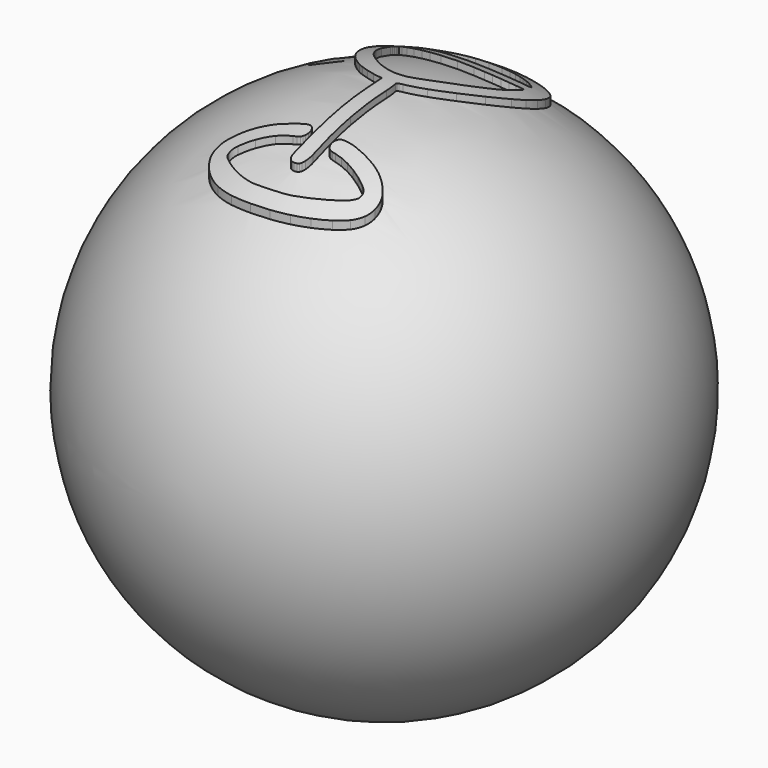
from build123d import *

# Parameters (mm, degrees)
F2_SCALE  = 33.3
F4_DEPTH  = 350
F5_SCALE  = 0.03
F8_SCALE  = 1.4
F9_R      = 2
F10_DEPTH = 25


# Not quite as in the source:
# - ends of sketch curves that miss each other by under 0.0002 mm in the source are joined


with BuildPart() as f1:
    # F0 (on Top) → F1 (revolve)
    with BuildSketch(Plane.XY):
        with BuildLine():
            ThreePointArc((0, 10), (-10, 0), (0, -10))
            Line((0, -10), (0, 10))
        make_face()
    revolve(axis=Axis((0, 0, 0), (0, 1, 0)))


with BuildPart() as f1_1:
    # F2: moved
    add(f1.part.scale(F2_SCALE))

    # F3 (on Top) → F4 (join)
    with BuildSketch(Plane.XY):
        with BuildLine():
            ThreePointArc((-17.0978460005, 193.3171829663), (-22.5521989544, 193.2279139935), (-27.9912949904, 192.8105779101))
            ThreePointArc((-27.9912949904, 192.8105779101), (-31.3832817791, 192.3903002928), (-34.7594609738, 191.8577388501))
            ThreePointArc((-34.7594609738, 191.8577388501), (-38.6008805736, 191.1421568562), (-42.4254231321, 190.3412595978))
            ThreePointArc((-42.4254231321, 190.3412595978), (-46.2931834784, 189.441445782), (-50.1401671634, 188.4565846103))
            ThreePointArc((-50.1401671634, 188.4565846103), (-53.618957919, 187.4704025999), (-57.0674972423, 186.3831507312))
            ThreePointArc((-57.0674972423, 186.3831507312), (-64.8016343565, 183.5621303497), (-72.3543253898, 180.28617383))
            ThreePointArc((-72.3543253898, 180.28617383), (-78.574954134, 176.996572469), (-84.4560219104, 173.1325408768))
            ThreePointArc((-84.4560219104, 173.1325408768), (-89.1434378782, 169.3023008105), (-93.3701958758, 164.9690428918))
            ThreePointArc((-93.3701958758, 164.9690428918), (-96.5854739254, 160.6281099929), (-99.0769773477, 155.8349771471))
            ThreePointArc((-99.0769773477, 155.8349771471), (-99.5068284417, 154.8258634849), (-99.9415123021, 153.8188221313))
            ThreePointArc((-99.9415123021, 153.8188221313), (-100.3930929277, 152.7857301658), (-100.8492287493, 151.7546413335))
            ThreePointArc((-100.8492287493, 151.7546413335), (-101.2599002155, 150.8372754179), (-101.6746101681, 149.9217280766))
            ThreePointArc((-101.6746101681, 149.9217280766), (-101.9531863531, 149.321958896), (-102.2404955652, 148.7263237863))
            ThreePointArc((-102.2404955652, 148.7263237863), (-102.5665518235, 147.8678723653), (-102.7268716663, 146.9636880546))
            ThreePointArc((-102.7268716663, 146.9636880546), (-102.820253294, 145.4142480108), (-102.8468239295, 143.8622240003))
            ThreePointArc((-102.8468239295, 143.8622240003), (-102.8017890764, 141.6009729286), (-102.6867114398, 139.3422029708))
            ThreePointArc((-102.6867114398, 139.3422029708), (-102.4440250928, 135.937420683), (-102.1689371991, 132.5351029829))
            ThreePointArc((-102.1689371991, 132.5351029829), (-100.0375071676, 114.1550624435), (-96.8073717537, 95.9359760513))
            ThreePointArc((-96.8073717537, 95.9359760513), (-92.9442600763, 81.5578835933), (-87.4706365699, 67.7125731991))
            ThreePointArc((-87.4706365699, 67.7125731991), (-81.1300528818, 56.1236300589), (-73.2948879198, 45.4879920679))
            ThreePointArc((-73.2948879198, 45.4879920679), (-63.9217794141, 35.7131224242), (-53.4058008805, 27.1798091677))
            ThreePointArc((-53.4058008805, 27.1798091677), (-49.2402137019, 24.4109552104), (-44.9025261202, 21.9203457739))
            ThreePointArc((-44.9025261202, 21.9203457739), (-39.8750977329, 19.3951162626), (-34.7367309001, 17.1040452387))
            ThreePointArc((-34.7367309001, 17.1040452387), (-29.5504863242, 15.0731835379), (-24.2757760482, 13.2846188463))
            ThreePointArc((-24.2757760482, 13.2846188463), (-19.621447429, 12.0050283954), (-14.8881420891, 11.0584834547))
            Line((-14.8881420891, 11.0584834547), (-11.28499, 10.469947))
            Line((-11.28499, 10.469947), (-10.560145, 2.237712))
            ThreePointArc((-10.560145, 2.237712), (-9.9476260486, -6.4407893964), (-9.6367378822, -15.1353229978))
            ThreePointArc((-9.6367378822, -15.1353229978), (-9.2911871236, -35.9008315673), (-9.0179850786, -56.6674180009))
            ThreePointArc((-9.0179850786, -56.6674180009), (-8.8229406584, -77.3194664112), (-8.7092667914, -97.9721229993))
            ThreePointArc((-8.7092667914, -97.9721229993), (-8.8098121517, -108.1744092953), (-9.1835099452, -118.3703450027))
            ThreePointArc((-9.1835099452, -118.3703450027), (-9.4747749065, -124.4063401519), (-9.7442124116, -130.4433490252))
            ThreePointArc((-9.7442124116, -130.4433490252), (-9.7789929679, -132.5732024208), (-9.7010406207, -134.701912976))
            ThreePointArc((-9.7010406207, -134.701912976), (-9.5228701649, -135.9359505595), (-9.1496069528, -137.1256009809))
            ThreePointArc((-9.1496069528, -137.1256009809), (-8.6038300896, -138.1821549577), (-7.87309221, -139.1203451973))
            ThreePointArc((-7.87309221, -139.1203451973), (-7.2722189346, -139.6998027787), (-6.6171708442, -140.2172307814))
            ThreePointArc((-6.6171708442, -140.2172307814), (-5.9618080364, -140.6252819631), (-5.2608069222, -140.9487067994))
            ThreePointArc((-5.2608069222, -140.9487067994), (-4.4831933039, -141.1997885004), (-3.6818591124, -141.3597528014))
            ThreePointArc((-3.6818591124, -141.3597528014), (-2.7188986466, -141.4607896854), (-1.75124, -141.494524))
            ThreePointArc((-1.75124, -141.494524), (-0.0066551217, -141.4167625272), (1.7240930059, -141.1840950327))
            ThreePointArc((1.7240930059, -141.1840950327), (3.0368774857, -140.8201904625), (4.2606372754, -140.2216574521))
            ThreePointArc((4.2606372754, -140.2216574521), (5.3148712932, -139.4296820141), (6.1963186971, -138.4490267768))
            ThreePointArc((6.1963186971, -138.4490267768), (7.0829288098, -137.1000522109), (7.8202605648, -135.6640328052))
            ThreePointArc((7.8202605648, -135.6640328052), (9.386626658, -130.8791872501), (9.9267429872, -125.873538))
            ThreePointArc((9.9267429872, -125.873538), (9.9733383312, -95.7774447642), (9.929765879, -65.6813470004))
            ThreePointArc((9.929765879, -65.6813470004), (9.7718961496, -36.7033266098), (9.4690230839, -7.7264589989))
            ThreePointArc((9.4690230839, -7.7264589989), (8.8939209502, 0.6968519395), (7.3940285242, 9.0054758867))
            ThreePointArc((7.3940285242, 9.0054758867), (7.3468365686, 9.5735728163), (7.4706734396, 10.1300128295))
            ThreePointArc((7.4706734396, 10.1300128295), (7.7532565447, 10.6138854213), (8.1727108229, 10.9854282785))
            ThreePointArc((8.1727108229, 10.9854282785), (8.9842439543, 11.4321716431), (9.8454969795, 11.7733590631))
            ThreePointArc((9.8454969795, 11.7733590631), (11.6722659814, 12.3491425642), (13.5089178367, 12.8925775705))
            ThreePointArc((13.5089178367, 12.8925775705), (25.5299883931, 17.3753752311), (36.7074171204, 23.6735258207))
            ThreePointArc((36.7074171204, 23.6735258207), (48.1911824499, 32.34457207), (58.6434100346, 42.2347109672))
            ThreePointArc((58.6434100346, 42.2347109672), (68.3554260068, 53.6702336239), (76.7924897103, 66.0762961751))
            ThreePointArc((76.7924897103, 66.0762961751), (83.5724843186, 78.9381773972), (88.7997903798, 92.5054758787))
            ThreePointArc((88.7997903798, 92.5054758787), (91.2346390502, 101.412003675), (92.9096409783, 110.4921520031))
            ThreePointArc((92.9096409783, 110.4921520031), (93.6739366176, 119.093603638), (93.5485160383, 127.7280340025))
            ThreePointArc((93.5485160383, 127.7280340025), (92.5566023081, 135.9260015333), (90.6817967179, 143.9681199179))
            ThreePointArc((90.6817967179, 143.9681199179), (87.9631422647, 151.6637080141), (84.3978090964, 159.0054760537))
            ThreePointArc((84.3978090964, 159.0054760537), (80.5955790543, 164.7521744689), (75.9651375367, 169.8551645673))
            ThreePointArc((75.9651375367, 169.8551645673), (70.2604730058, 174.632045463), (64.0200449693, 178.6840629458))
            ThreePointArc((64.0200449693, 178.6840629458), (56.4813674028, 182.446779857), (48.5907810902, 185.4011572857))
            ThreePointArc((48.5907810902, 185.4011572857), (39.2556829448, 187.9986899339), (29.7635968656, 189.9458762068))
            ThreePointArc((29.7635968656, 189.9458762068), (23.2428353504, 190.9151557052), (16.688195058, 191.6198006659))
            ThreePointArc((16.688195058, 191.6198006659), (8.1312124486, 192.2845679193), (-0.436677962, 192.7896627665))
            ThreePointArc((-0.436677962, 192.7896627665), (-8.7649000272, 193.1280228025), (-17.0978460005, 193.3171829663))
        make_face()
        with BuildLine():
            ThreePointArc((74.4088944707, 123.7898260105), (74.4467436235, 121.3518755172), (74.4515614652, 118.9136359978))
            ThreePointArc((74.4515614652, 118.9136359978), (74.2079240991, 112.8985314954), (73.5359877974, 106.9161120301))
            ThreePointArc((73.5359877974, 106.9161120301), (72.4706715951, 101.4582625361), (70.9166328231, 96.1189757195))
            ThreePointArc((70.9166328231, 96.1189757195), (68.7880576441, 90.6377106911), (66.2076911137, 85.3540749384))
            ThreePointArc((66.2076911137, 85.3540749384), (62.7251090021, 79.2902245988), (58.9429106921, 73.4085892091))
            ThreePointArc((58.9429106921, 73.4085892091), (54.7160561513, 67.6664487294), (50.065401769, 62.2618312145))
            ThreePointArc((50.065401769, 62.2618312145), (44.3662373256, 56.4317729664), (38.3774171127, 50.8996768715))
            ThreePointArc((38.3774171127, 50.8996768715), (32.0999551252, 45.6674505647), (25.5643739269, 40.7614441027))
            ThreePointArc((25.5643739269, 40.7614441027), (19.5553828747, 36.8144375608), (13.2689679142, 33.3261971691))
            ThreePointArc((13.2689679142, 33.3261971691), (10.863301237, 32.1425066895), (8.4298508589, 31.0170403149))
            ThreePointArc((8.4298508589, 31.0170403149), (6.7506726676, 30.3385795546), (5.0257309816, 29.786742066))
            ThreePointArc((5.0257309816, 29.786742066), (3.3264109283, 29.3840013041), (1.6004799119, 29.1174477726))
            ThreePointArc((1.6004799119, 29.1174477726), (-0.8122032121, 28.8798180191), (-3.231032039, 28.7161877456))
            ThreePointArc((-3.231032039, 28.7161877456), (-5.588666528, 28.6256661874), (-7.9479040026, 28.6005031721))
            ThreePointArc((-7.9479040026, 28.6005031721), (-9.6922083492, 28.6643607632), (-11.4283590028, 28.8445169794))
            ThreePointArc((-11.4283590028, 28.8445169794), (-13.1537951105, 29.1407539805), (-14.8557462129, 29.5509352301))
            ThreePointArc((-14.8557462129, 29.5509352301), (-17.1395206186, 30.2158571345), (-19.4043827895, 30.9425936267))
            ThreePointArc((-19.4043827895, 30.9425936267), (-24.2924915898, 32.7737492249), (-29.0433831163, 34.9361017661))
            ThreePointArc((-29.0433831163, 34.9361017661), (-33.8455310473, 37.5079887033), (-38.4835330177, 40.3652889731))
            ThreePointArc((-38.4835330177, 40.3652889731), (-43.2852405931, 43.7232093014), (-47.8922237345, 47.3436693191))
            ThreePointArc((-47.8922237345, 47.3436693191), (-52.7565526798, 51.5669384943), (-57.4391437184, 55.9908552858))
            ThreePointArc((-57.4391437184, 55.9908552858), (-62.2307975599, 61.1677128001), (-66.5265149619, 66.7629440265))
            ThreePointArc((-66.5265149619, 66.7629440265), (-70.151615065, 72.5661984631), (-73.1743823077, 78.7047642986))
            ThreePointArc((-73.1743823077, 78.7047642986), (-75.8907685733, 85.8410453159), (-77.9773704047, 93.1862039038))
            ThreePointArc((-77.9773704047, 93.1862039038), (-79.9537267091, 102.4451536476), (-81.5017276344, 111.7852729098))
            ThreePointArc((-81.5017276344, 111.7852729098), (-81.7871031173, 113.8397072827), (-82.0593620766, 115.8959209901))
            ThreePointArc((-82.0593620766, 115.8959209901), (-82.3036275829, 117.8447110628), (-82.5332391841, 119.795281979))
            ThreePointArc((-82.5332391841, 119.795281979), (-82.7154817286, 121.4436107109), (-82.8868350178, 123.0931069982))
            ThreePointArc((-82.8868350178, 123.0931069982), (-82.9486906346, 123.896354978), (-82.972974873, 124.7016150009))
            Line((-82.972974873, 124.7016150009), (-82.991295, 127.397753))
            Line((-82.991295, 127.397753), (-77.241295, 125.412895))
            ThreePointArc((-77.241295, 125.412895), (-73.456347914, 124.2169391025), (-69.6136839641, 123.2219171553))
            ThreePointArc((-69.6136839641, 123.2219171553), (-64.0875525023, 122.0000367541), (-58.5393610614, 120.8825876794))
            ThreePointArc((-58.5393610614, 120.8825876794), (-52.5523505329, 119.7941436789), (-46.5457790369, 118.819410758))
            ThreePointArc((-46.5457790369, 118.819410758), (-41.1095909133, 118.0617088649), (-35.6556589677, 117.4445543223))
            ThreePointArc((-35.6556589677, 117.4445543223), (-28.2576291485, 116.8706183037), (-20.8413430001, 116.627826988))
            ThreePointArc((-20.8413430001, 116.627826988), (-10.3942850651, 116.605941948), (0.0517019887, 116.7571134976))
            ThreePointArc((0.0517019887, 116.7571134976), (10.2994367513, 117.0706979467), (20.5409970004, 117.5448779927))
            ThreePointArc((20.5409970004, 117.5448779927), (26.7977594297, 118.0806794205), (33.0087050428, 119.0071317641))
            ThreePointArc((33.0087050428, 119.0071317641), (37.4770940187, 119.8754409899), (41.9223120051, 120.8554909781))
            ThreePointArc((41.9223120051, 120.8554909781), (46.3327123246, 121.9448277229), (50.7142390819, 123.1450397151))
            ThreePointArc((50.7142390819, 123.1450397151), (54.8114636035, 124.3819911316), (58.8745489881, 125.7268460344))
            ThreePointArc((58.8745489881, 125.7268460344), (62.3972920001, 127.0224241863), (65.8666769199, 128.4547681837))
            ThreePointArc((65.8666769199, 128.4547681837), (67.1708233931, 129.0105552399), (68.4839450211, 129.5447919469))
            ThreePointArc((68.4839450211, 129.5447919469), (69.6625458679, 129.9972152018), (70.8513591187, 130.4220796554))
            ThreePointArc((70.8513591187, 130.4220796554), (71.8435308202, 130.7549523068), (72.8408398861, 131.0721013681))
            ThreePointArc((72.8408398861, 131.0721013681), (73.1737949102, 131.1259739019), (73.5087049961, 131.0860179854))
            ThreePointArc((73.5087049961, 131.0860179854), (73.7992903483, 130.9044343175), (73.9364649931, 130.5904349992))
            ThreePointArc((73.9364649931, 130.5904349992), (74.0899957249, 129.1063261903), (74.2179988774, 127.619798068))
            ThreePointArc((74.2179988774, 127.619798068), (74.3397810335, 125.7061246083), (74.4088944707, 123.7898260105))
        make_face(mode=Mode.SUBTRACT)
        with BuildLine():
            ThreePointArc((12.1078240022, 173.204657039), (17.5742671841, 172.7462077487), (23.0080560003, 171.9938010016))
            ThreePointArc((23.0080560003, 171.9938010016), (27.2734206987, 171.2409668581), (31.5226340335, 170.4017521609))
            ThreePointArc((31.5226340335, 170.4017521609), (34.900508384, 169.6295480334), (38.2455080109, 168.7254950375))
            ThreePointArc((38.2455080109, 168.7254950375), (41.2783072399, 167.7685323892), (44.2659140375, 166.6786450962))
            ThreePointArc((44.2659140375, 166.6786450962), (47.4344506878, 165.3778505212), (50.555022307, 163.9658576478))
            ThreePointArc((50.555022307, 163.9658576478), (53.4355806501, 162.4736282241), (56.2034280202, 160.7814740306))
            ThreePointArc((56.2034280202, 160.7814740306), (59.0524811445, 158.7786357365), (61.7823132676, 156.6161183187))
            ThreePointArc((61.7823132676, 156.6161183187), (64.0782257508, 154.5985751733), (66.2815546756, 152.4803126773))
            ThreePointArc((66.2815546756, 152.4803126773), (66.8378890025, 151.4784912745), (66.7867613291, 150.3337032226))
            ThreePointArc((66.7867613291, 150.3337032226), (66.1203790019, 149.1898539304), (65.0499871785, 148.4109326024))
            ThreePointArc((65.0499871785, 148.4109326024), (60.7924254224, 146.5458677211), (56.5016636547, 144.7585058505))
            ThreePointArc((56.5016636547, 144.7585058505), (51.7428602635, 142.9141478929), (46.9279311091, 141.2217166732))
            ThreePointArc((46.9279311091, 141.2217166732), (42.3415981533, 139.7872309663), (37.7040670082, 138.5280629672))
            ThreePointArc((37.7040670082, 138.5280629672), (24.8338411606, 135.838854263), (11.7894239192, 134.1902989424))
            ThreePointArc((11.7894239192, 134.1902989424), (-2.0674194935, 133.477244859), (-15.9406120037, 133.711948927))
            ThreePointArc((-15.9406120037, 133.711948927), (-29.7251636597, 134.8910760058), (-43.3966739149, 137.0109844474))
            ThreePointArc((-43.3966739149, 137.0109844474), (-56.0863915319, 139.9696876023), (-68.4912951883, 143.9573214872))
            ThreePointArc((-68.4912951883, 143.9573214872), (-70.451900958, 144.6764891053), (-72.4131289898, 145.393958028))
            ThreePointArc((-72.4131289898, 145.393958028), (-74.1666695628, 146.0333872436), (-75.9209827759, 146.670693618))
            ThreePointArc((-75.9209827759, 146.670693618), (-77.4001688481, 147.2064365098), (-78.8797400241, 147.7411149333))
            ThreePointArc((-78.8797400241, 147.7411149333), (-79.3093275416, 147.8922831568), (-79.741294756, 148.0365107508))
            ThreePointArc((-79.741294756, 148.0365107508), (-80.2531229337, 148.3195670983), (-80.6225632322, 148.7730018754))
            ThreePointArc((-80.6225632322, 148.7730018754), (-80.7373417468, 149.2762491892), (-80.5785603943, 149.767391259))
            ThreePointArc((-80.5785603943, 149.767391259), (-79.9436571793, 150.5965336499), (-79.1958301107, 151.3254601314))
            ThreePointArc((-79.1958301107, 151.3254601314), (-77.4818155528, 152.7423655701), (-75.7412945538, 154.126581428))
            ThreePointArc((-75.7412945538, 154.126581428), (-70.7640863277, 157.7619229289), (-65.5674757672, 161.0760666083))
            ThreePointArc((-65.5674757672, 161.0760666083), (-60.0839156253, 164.1158318847), (-54.4280328796, 166.8214917277))
            ThreePointArc((-54.4280328796, 166.8214917277), (-48.7746147087, 169.1156092494), (-42.9909770288, 171.0581970953))
            ThreePointArc((-42.9909770288, 171.0581970953), (-37.5075223126, 172.487511331), (-31.9307199487, 173.4927426358))
            ThreePointArc((-31.9307199487, 173.4927426358), (-27.167726513, 173.9950904892), (-22.3812849998, 174.1637242115))
            ThreePointArc((-22.3812849998, 174.1637242115), (-13.7889609334, 174.1069727121), (-5.198234986, 173.9318115126))
            ThreePointArc((-5.198234986, 173.9318115126), (3.4574696998, 173.6319029966), (12.1078240022, 173.204657039))
        make_face(mode=Mode.SUBTRACT)
        with BuildLine():
            ThreePointArc((-25.6309609606, -94.2784421714), (-30.1490997281, -95.3523380113), (-34.6507459555, -96.4933951702))
            ThreePointArc((-34.6507459555, -96.4933951702), (-43.4652886859, -99.009449081), (-52.1585541286, -101.9169956422))
            ThreePointArc((-52.1585541286, -101.9169956422), (-59.9986625299, -104.9933371149), (-67.6486410799, -108.5159788389))
            ThreePointArc((-67.6486410799, -108.5159788389), (-74.3299010912, -112.0989578101), (-80.769079775, -116.1007013376))
            ThreePointArc((-80.769079775, -116.1007013376), (-86.1431534637, -120.0571886864), (-91.1251584237, -124.4972435671))
            ThreePointArc((-91.1251584237, -124.4972435671), (-93.2603279824, -126.6267506745), (-95.3547942343, -128.796303778))
            ThreePointArc((-95.3547942343, -128.796303778), (-96.5938454052, -130.2035437895), (-97.7272761932, -131.6971658642))
            ThreePointArc((-97.7272761932, -131.6971658642), (-98.5561982293, -133.0122237947), (-99.2488042217, -134.4039083397))
            ThreePointArc((-99.2488042217, -134.4039083397), (-99.9181196115, -136.0829354383), (-100.4782020074, -137.8014879978))
            ThreePointArc((-100.4782020074, -137.8014879978), (-101.1020611523, -140.4921143342), (-101.4263804881, -143.2350119694))
            ThreePointArc((-101.4263804881, -143.2350119694), (-101.4110471487, -145.8009307626), (-101.0449314656, -148.3406421001))
            ThreePointArc((-101.0449314656, -148.3406421001), (-100.2935863365, -151.0265240879), (-99.2209593802, -153.6010051864))
            ThreePointArc((-99.2209593802, -153.6010051864), (-97.6120855463, -156.6244865396), (-95.8058502385, -159.5343711593))
            ThreePointArc((-95.8058502385, -159.5343711593), (-89.9230710064, -166.9417662427), (-82.9046506524, -173.283561545))
            ThreePointArc((-82.9046506524, -173.283561545), (-74.3166883243, -179.0204343497), (-65.0717090139, -183.6242550329))
            ThreePointArc((-65.0717090139, -183.6242550329), (-54.0161686364, -187.5847586679), (-42.5949349897, -190.3171539435))
            ThreePointArc((-42.5949349897, -190.3171539435), (-29.2888044037, -192.2431378788), (-15.8776539913, -193.1937007459))
            ThreePointArc((-15.8776539913, -193.1937007459), (-3.5960486329, -193.2791801199), (8.6719109775, -192.6941127008))
            ThreePointArc((8.6719109775, -192.6941127008), (20.3021983256, -191.4499798602), (31.830659933, -189.4736136719))
            ThreePointArc((31.830659933, -189.4736136719), (42.8221670835, -186.8513395493), (53.6180930111, -183.5140450322))
            ThreePointArc((53.6180930111, -183.5140450322), (63.9937540235, -179.524640278), (74.0700660274, -174.8302150539))
            ThreePointArc((74.0700660274, -174.8302150539), (81.8920325619, -170.3636990635), (89.2457368561, -165.1621648161))
            ThreePointArc((89.2457368561, -165.1621648161), (94.5537890315, -160.1730258829), (98.8780632953, -154.3106391791))
            ThreePointArc((98.8780632953, -154.3106391791), (101.475983583, -148.6670746711), (102.734546657, -142.583076969))
            ThreePointArc((102.734546657, -142.583076969), (102.593996748, -136.3556140946), (101.0635003023, -130.3175158859))
            ThreePointArc((101.0635003023, -130.3175158859), (99.794333154, -127.5554693211), (98.153979935, -124.9963820483))
            ThreePointArc((98.153979935, -124.9963820483), (95.7992341868, -122.0657377619), (93.233131867, -119.3182621338))
            ThreePointArc((93.233131867, -119.3182621338), (90.2491227697, -116.5549142564), (87.0776710209, -114.008878972))
            ThreePointArc((87.0776710209, -114.008878972), (83.8135447689, -111.7612568415), (80.3876579098, -109.7688651697))
            ThreePointArc((80.3876579098, -109.7688651697), (74.8015095412, -107.0565811371), (69.0318911145, -104.7602706786))
            ThreePointArc((69.0318911145, -104.7602706786), (62.0645346051, -102.4522560207), (55.0012739518, -100.4569271864))
            ThreePointArc((55.0012739518, -100.4569271864), (47.945004804, -98.7996856782), (40.8217130521, -97.4594996842))
            ThreePointArc((40.8217130521, -97.4594996842), (34.9566168238, -96.7361748219), (29.052029, -96.494524))
            ThreePointArc((29.052029, -96.494524), (27.1383256532, -96.5168823103), (25.2256670004, -96.583944008))
            ThreePointArc((25.2256670004, -96.583944008), (24.1470552283, -96.6960244136), (23.0881051591, -96.9296695663))
            ThreePointArc((23.0881051591, -96.9296695663), (22.2772488999, -97.235121139), (21.5308961641, -97.6752872303))
            ThreePointArc((21.5308961641, -97.6752872303), (20.7093400282, -98.32418137), (19.9557459915, -99.050895992))
            ThreePointArc((19.9557459915, -99.050895992), (18.9080995735, -100.4137559543), (18.1484472786, -101.9557931045))
            ThreePointArc((18.1484472786, -101.9557931045), (17.6690011719, -103.6799422217), (17.4977408472, -105.4612980069))
            ThreePointArc((17.4977408472, -105.4612980069), (17.6401779372, -107.2344482358), (18.091960421, -108.9549838487))
            ThreePointArc((18.091960421, -108.9549838487), (18.8243614067, -110.4814030715), (19.8515448924, -111.8272341011))
            ThreePointArc((19.8515448924, -111.8272341011), (20.5830684705, -112.51476038), (21.394251034, -113.1062009468))
            ThreePointArc((21.394251034, -113.1062009468), (22.2598955337, -113.5819186852), (23.1801148733, -113.9408674))
            ThreePointArc((23.1801148733, -113.9408674), (24.4301076552, -114.2790771878), (25.7042450237, -114.510251828))
            ThreePointArc((25.7042450237, -114.510251828), (27.76388531, -114.7711192494), (29.8288169346, -114.9861247043))
            ThreePointArc((29.8288169346, -114.9861247043), (34.3797446015, -115.5247239199), (38.8978029327, -116.291653344))
            ThreePointArc((38.8978029327, -116.291653344), (43.6588417664, -117.3276791308), (48.3723078471, -118.5622145377))
            ThreePointArc((48.3723078471, -118.5622145377), (53.1325870319, -120.0225298781), (57.8288569272, -121.6771681939))
            ThreePointArc((57.8288569272, -121.6771681939), (62.3787337627, -123.4988762485), (66.8459152255, -125.5148845277))
            ThreePointArc((66.8459152255, -125.5148845277), (71.0948431859, -127.6102300887), (75.2892890445, -129.8126119178))
            ThreePointArc((75.2892890445, -129.8126119178), (77.6600838674, -131.2739338162), (79.8520057627, -132.99195827))
            ThreePointArc((79.8520057627, -132.99195827), (81.1740872568, -134.4148275357), (82.1834367359, -136.074246126))
            ThreePointArc((82.1834367359, -136.074246126), (82.7998083216, -137.8504505031), (83.008705, -139.71892))
            ThreePointArc((83.008705, -139.71892), (82.957288215, -140.8273209909), (82.8034800294, -141.9262020055))
            ThreePointArc((82.8034800294, -141.9262020055), (82.5613043654, -142.8209731266), (82.181521264, -143.6665671446))
            ThreePointArc((82.181521264, -143.6665671446), (81.5982556062, -144.5975498383), (80.9100574098, -145.4538854658))
            ThreePointArc((80.9100574098, -145.4538854658), (79.7254057044, -146.7214002917), (78.5007796116, -147.9503366292))
            ThreePointArc((78.5007796116, -147.9503366292), (74.2194912714, -151.5839455246), (69.4887517998, -154.6092796349))
            ThreePointArc((69.4887517998, -154.6092796349), (62.2331929435, -158.374835051), (54.813210218, -161.8050535014))
            ThreePointArc((54.813210218, -161.8050535014), (46.4739058362, -165.2092427039), (37.9891800946, -168.2328052856))
            ThreePointArc((37.9891800946, -168.2328052856), (29.8832603682, -170.6734754852), (21.6564680984, -172.6691444602))
            ThreePointArc((21.6564680984, -172.6691444602), (15.5949660919, -173.7476301695), (9.4733170066, -174.4036410919))
            ThreePointArc((9.4733170066, -174.4036410919), (1.4369201244, -174.8566039811), (-6.6097710041, -175.0556315432))
            ThreePointArc((-6.6097710041, -175.0556315432), (-14.5657951772, -175.0021169994), (-22.5162369896, -174.6993638064))
            ThreePointArc((-22.5162369896, -174.6993638064), (-28.2762899332, -174.1601076225), (-33.9755861208, -173.1666135606))
            ThreePointArc((-33.9755861208, -173.1666135606), (-42.0895701192, -171.0709214736), (-50.0070901361, -168.3247353463))
            ThreePointArc((-50.0070901361, -168.3247353463), (-57.9453586228, -164.8634144819), (-65.6079723713, -160.8284176464))
            ThreePointArc((-65.6079723713, -160.8284176464), (-71.869342165, -156.9323919415), (-77.8414560392, -152.6060050503))
            ThreePointArc((-77.8414560392, -152.6060050503), (-80.1617569167, -149.7456147077), (-80.991295, -146.157092))
            ThreePointArc((-80.991295, -146.157092), (-79.936828628, -141.3041391968), (-76.9635820316, -137.3263439636))
            ThreePointArc((-76.9635820316, -137.3263439636), (-69.9987322145, -131.7893299522), (-62.5812439869, -126.8752150217))
            ThreePointArc((-62.5812439869, -126.8752150217), (-53.5995666966, -121.9850030543), (-44.2290187381, -117.8889646776))
            ThreePointArc((-44.2290187381, -117.8889646776), (-35.2427919156, -114.9701311433), (-25.9912950042, -113.0513639718))
            ThreePointArc((-25.9912950042, -113.0513639718), (-23.7160381834, -112.6560074023), (-21.4606950511, -112.1594917903))
            ThreePointArc((-21.4606950511, -112.1594917903), (-19.8271321965, -111.6666885865), (-18.2561710897, -111.0007578167))
            ThreePointArc((-18.2561710897, -111.0007578167), (-17.074055272, -110.311096436), (-16.0052287448, -109.4563212752))
            ThreePointArc((-16.0052287448, -109.4563212752), (-15.1357337669, -108.4974624009), (-14.4441366943, -107.4033301581))
            ThreePointArc((-14.4441366943, -107.4033301581), (-13.7624896817, -105.8566886874), (-13.2777989727, -104.2374860063))
            ThreePointArc((-13.2777989727, -104.2374860063), (-13.0451928037, -102.6956153806), (-13.0580478506, -101.1363509869))
            ThreePointArc((-13.0580478506, -101.1363509869), (-13.3098342858, -99.6927408941), (-13.8034596389, -98.3129798348))
            ThreePointArc((-13.8034596389, -98.3129798348), (-14.5190649244, -97.0576669001), (-15.4458401033, -95.9490691033))
            ThreePointArc((-15.4458401033, -95.9490691033), (-16.6513897544, -94.9631110176), (-18.0285942501, -94.2359446156))
            ThreePointArc((-18.0285942501, -94.2359446156), (-19.5060729867, -93.8073045627), (-21.0401220117, -93.6916775885))
            ThreePointArc((-21.0401220117, -93.6916775885), (-23.3500445003, -93.8715885924), (-25.6309609606, -94.2784421714))
        make_face()
    extrude(amount=F4_DEPTH)


with BuildPart() as f1_2:
    # F5: moved
    add(f1_1.part.scale(F5_SCALE))

    # F6 (on Top) → F7 (revolve, cut)
    with BuildSketch(Plane.XY):
        with BuildLine():
            Line((0, 10.25), (0, 15))
            ThreePointArc((0, 15), (-15, 0), (0, -15))
            Line((0, -15), (0, -10.25))
            ThreePointArc((0, -10.25), (-10.25, 0), (0, 10.25))
        make_face()
        with BuildLine():
            Line((0, -7), (0, 7))
            ThreePointArc((0, 7), (-7, 0), (0, -7))
        make_face()
    revolve(axis=Axis((0, 0, 0), (0, -1, 0)), mode=Mode.SUBTRACT)


with BuildPart() as f1_3:
    # F8: moved
    add(f1_2.part.scale(F8_SCALE))

    # F9 (on Front) → F10 (cut)
    with BuildSketch(Plane.XZ):
        with Locations((0, -5.1200183504)):
            Circle(F9_R)
    extrude(amount=-F10_DEPTH, mode=Mode.SUBTRACT)


solid = f1_3.part
